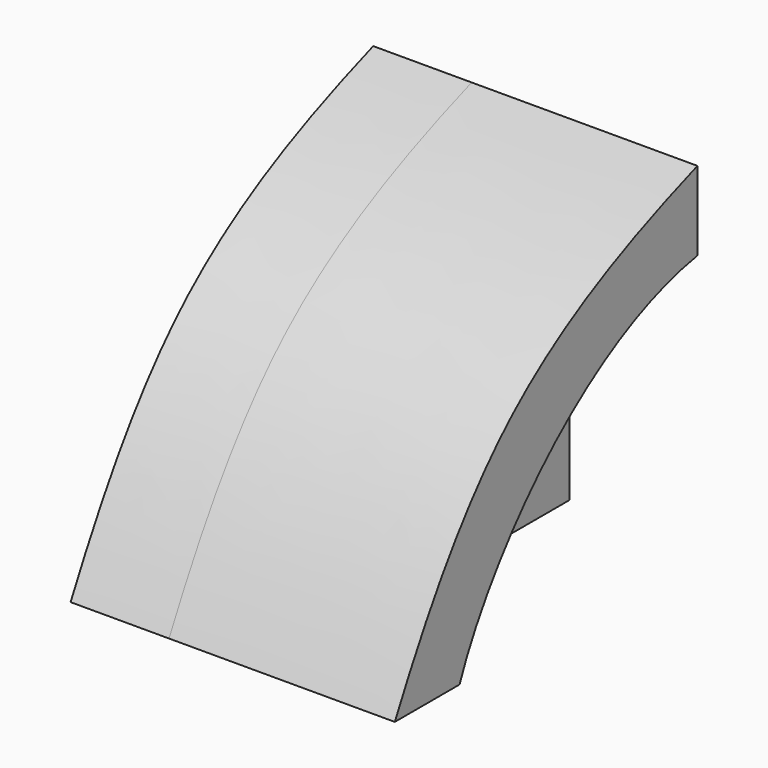
from build123d import *

# Parameters (mm, degrees)
F3_DEPTH      = 5.075
F4_DEPTH      = 11.7
F4_DEPTH_BACK = 5.1


# Not quite as in the source:
# - the program builds the solid bodies; features that only make, move or delete a surface that nothing else refers to are left out


with BuildPart() as f3:
    # F2 (on Right) → F3 (new body, symmetric)
    with BuildSketch(Plane.YZ):
        with BuildLine():
            Line((-28.3462911332, -4.9449687588), (-28.3462911332, 8.3612054586))
            add(Edge.make_bspline(
                [(-43.7509737622, -4.9449687588), (-41.7884092148, 0), (-35.7711096695, 7.1036480367), (-28.3462911332, 8.3612054586)],
                knots=[0, 0, 0, 0, 20.3557981716, 20.3557981716, 20.3557981716, 20.3557981716], degree=3))
            Line((-43.7509737622, -4.9449687588), (-28.3462911332, -4.9449687588))
        make_face()
    extrude(amount=F3_DEPTH, both=True)

    # F2 (on Right) → F4 (join, two sides)
    with BuildSketch(Plane.YZ) as f4_sk:
        with BuildLine():
            Line((-28.3462911332, 8.3612054586), (-28.3462911332, 12.4550312412))
            add(Edge.make_bspline(
                [(-47.9462911332, -4.9449687588), (-46.2080227994, -1.5012717921), (-41.5989810613, 6.6616658975), (-33.5069069781, 10.6230272322), (-28.3462911332, 12.4550312412)],
                knots=[0, 0, 0, 0, 0.4814819879, 1, 1, 1, 1], degree=3))
            Line((-47.9462911332, -4.9449687588), (-43.7509737622, -4.9449687588))
            add(Edge.make_bspline(
                [(-43.7509737622, -4.9449687588), (-41.7884092148, 0), (-35.7711096695, 7.1036480367), (-28.3462911332, 8.3612054586)],
                knots=[0, 0, 0, 0, 20.3557981716, 20.3557981716, 20.3557981716, 20.3557981716], degree=3))
        make_face()
    extrude(amount=F4_DEPTH)
    extrude(f4_sk.sketch, amount=-F4_DEPTH_BACK)


solid = f3.part
